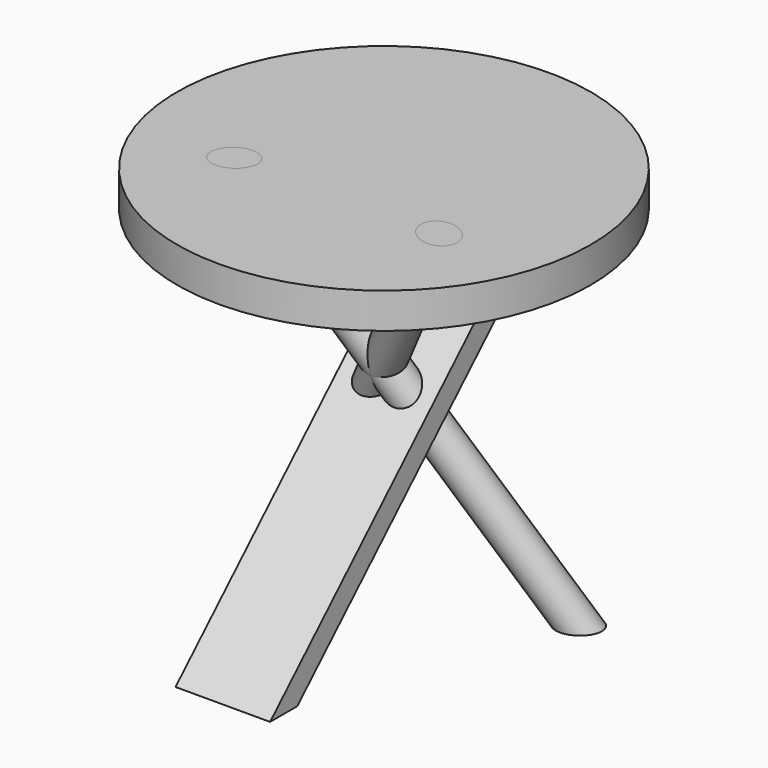
from build123d import *

# Parameters (mm, degrees)
F0_W           = 80
F0_H           = 300.734500748
F0_H_2         = 20
F1_DEPTH       = 30
F4_DEPTH       = 40
F8_R           = 15
F9_DEPTH       = 481.7550188272
F10_DEPTH      = 481.7550188272
F11_DEPTH      = 481.7550188272
F11_DEPTH_BACK = 50
F13_DEPTH      = 49.5977982638
F14_W          = 425
F14_H          = 300
F15_DEPTH      = 73.8088242034
F20_R          = 15
F21_REACH      = 574.1814256984
F23_DEPTH      = 49.5977982638


with BuildPart() as f1:
    # F0 (on Top) → F1 (new body)
    with BuildSketch(Plane.XY):
        with BuildLine():
            Line((-40, 150.367250374), (-40, 170.367250374))
            ThreePointArc((-40, 170.367250374), (-175, 0), (-40, -170.367250374))
            Line((-40, -170.367250374), (-40, -150.367250374))
            Line((-40, -150.367250374), (-40, 150.367250374))
        make_face()
        Rectangle(F0_W, F0_H)
        with Locations((0, 160.367250374)):
            Rectangle(F0_W, F0_H_2)
        with BuildLine():
            Line((-40, 170.367250374), (40, 170.367250374))
            ThreePointArc((40, 170.367250374), (0, 175), (-40, 170.367250374))
        make_face()
        with BuildLine():
            ThreePointArc((40, -170.367250374), (137.1586672435, -108.6853255964), (175, 0))
            ThreePointArc((175, 0), (137.1586672435, 108.6853255964), (40, 170.367250374))
            Line((40, 170.367250374), (40, 150.367250374))
            Line((40, 150.367250374), (40, -150.367250374))
            Line((40, -150.367250374), (40, -170.367250374))
        make_face()
        with Locations((0, -160.367250374)):
            Rectangle(F0_W, F0_H_2)
        with BuildLine():
            ThreePointArc((-40, -170.367250374), (0, -175), (40, -170.367250374))
            Line((40, -170.367250374), (-40, -170.367250374))
        make_face()
    extrude(amount=F1_DEPTH)


with BuildPart() as f4:
    # F3 (on Right) → F4 (new body, symmetric)
    with BuildSketch(Plane.YZ):
        Polygon((170.367250374, 2.1576976805), (170.367250374, 30), (-170.367250374, -300), (-141.6192716452, -300), align=None)
    extrude(amount=F4_DEPTH, both=True)


with BuildPart() as f9_tool:
    # F8 (on line) → F9 (new body, through all)
    with BuildSketch(Plane(origin=(-158.6839007787, 91.6161928307, -262.8986402967), x_dir=(0.8687864318, 0.1629539008, -0.4676068457), z_dir=(-0.4951869707, 0.2858963308, -0.8203981668))):
        with Locations((53.0632116259, 37.3429156197)):
            Circle(F8_R)
    extrude(amount=-F9_DEPTH)


with BuildPart() as f1_1:
    add(f1.part)

    # F9: cut by f9_tool
    add(f9_tool.part, mode=Mode.SUBTRACT)

    # F8 (on line) → F10 (cut, through all)
    with BuildSketch(Plane(origin=(-158.6839007787, 91.6161928307, -262.8986402967), x_dir=(0.8687864318, 0.1629539008, -0.4676068457), z_dir=(-0.4951869707, 0.2858963308, -0.8203981668))):
        with Locations((53.0632116259, 37.3429156197)):
            Circle(F8_R)
    extrude(amount=-F10_DEPTH, mode=Mode.SUBTRACT)


with BuildPart() as f4_1:
    add(f4.part)

    # F9: cut by f9_tool
    add(f9_tool.part, mode=Mode.SUBTRACT)


with BuildPart() as f11:
    # F8 (on line) → F11 (new body, two sides)
    with BuildSketch(Plane(origin=(-158.6839007787, 91.6161928307, -262.8986402967), x_dir=(0.8687864318, 0.1629539008, -0.4676068457), z_dir=(-0.4951869707, 0.2858963308, -0.8203981668))) as f11_sk:
        with Locations((53.0632116259, 37.3429156197)):
            Circle(F8_R)
    extrude(amount=-F11_DEPTH)
    extrude(f11_sk.sketch, amount=F11_DEPTH_BACK)

    # F12 (on face) → F13 (cut, through all)
    with BuildSketch(Plane(origin=(0, 0, -300), x_dir=(1, 0, 0), z_dir=(0, 0, -1))):
        Polygon((-40, 141.6192716452), (-40, 170.367250374), (-160, 170.367250374), (-160, -119.632749626), (40, -119.632749626), (40, 141.6192716452), align=None)
    extrude(amount=F13_DEPTH, mode=Mode.SUBTRACT)

    # F14 (on face) → F15 (cut, through all)
    with BuildSketch(Plane.XY.offset(30)):
        Rectangle(F14_W, F14_H)
    extrude(amount=F15_DEPTH, mode=Mode.SUBTRACT)


with BuildPart() as f21:
    f21_end = f1_1.part.faces().sort_by_distance((-0.7825626972, 0.4518127839, 30))[0]
    # F20 (on line) → F21 (new body, up to a face of F1 that its end follows)
    with BuildSketch(Plane(origin=(183.4432493147, 105.9110093729, -303.9185486352), x_dir=(0.8687864318, -0.1629539008, 0.4676068457), z_dir=(0.4951869707, 0.2858963308, -0.8203981668))):
        with Locations((-53.0632116259, 37.3429156197)):
            Circle(F20_R)
    f21_long = extrude(amount=-F21_REACH, mode=Mode.PRIVATE)
    add(split(f21_long, bisect_by=f21_end, keep=Keep.BOTTOM, mode=Mode.PRIVATE))

    # F22 (on face) → F23 (cut, through all)
    with BuildSketch(Plane(origin=(0, 0, -300), x_dir=(1, 0, 0), z_dir=(0, 0, -1))):
        Polygon((260, 170.367250374), (40, 170.367250374), (40, 141.6192716452), (-40, 141.6192716452), (-40, -129.632749626), (260, -129.632749626), align=None)
    extrude(amount=F23_DEPTH, mode=Mode.SUBTRACT)


solid = Compound([f1_1.part, f4_1.part, f11.part, f21.part])
